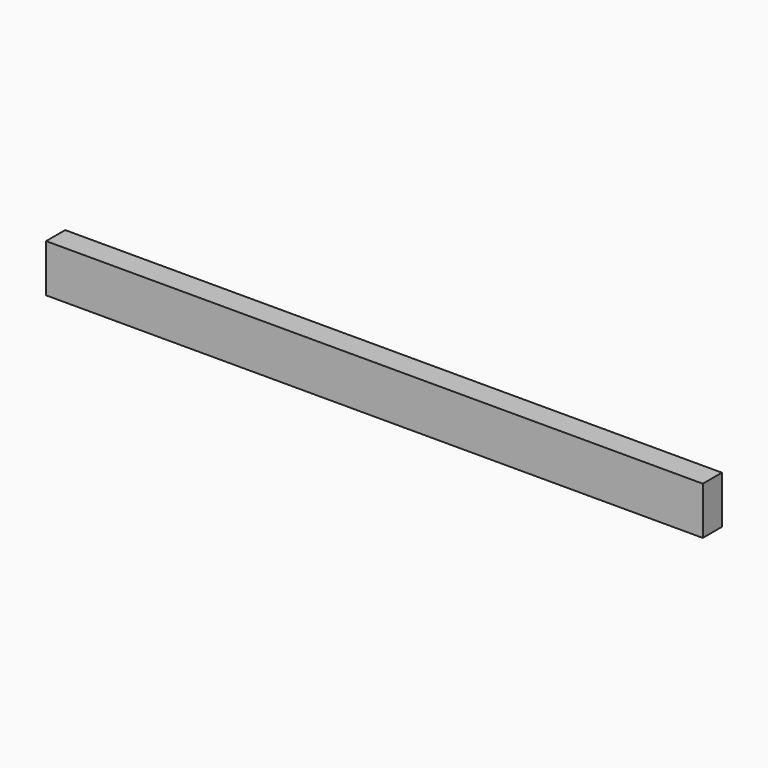
from build123d import *

# Parameters (mm, degrees)
F0_W     = 1100
F0_H     = 80
F1_DEPTH = 20
F2_ANGLE = 90


with BuildPart() as f1:
    # F0 (on Top) → F1 (new body, symmetric)
    with BuildSketch(Plane.XY):
        Rectangle(F0_W, F0_H)
    extrude(amount=F1_DEPTH, both=True)


with BuildPart() as f1_1:
    # F2: moved
    add(f1.part.rotate(Axis((0, -40, -20), (1, 0, 0)), F2_ANGLE))


solid = f1_1.part
